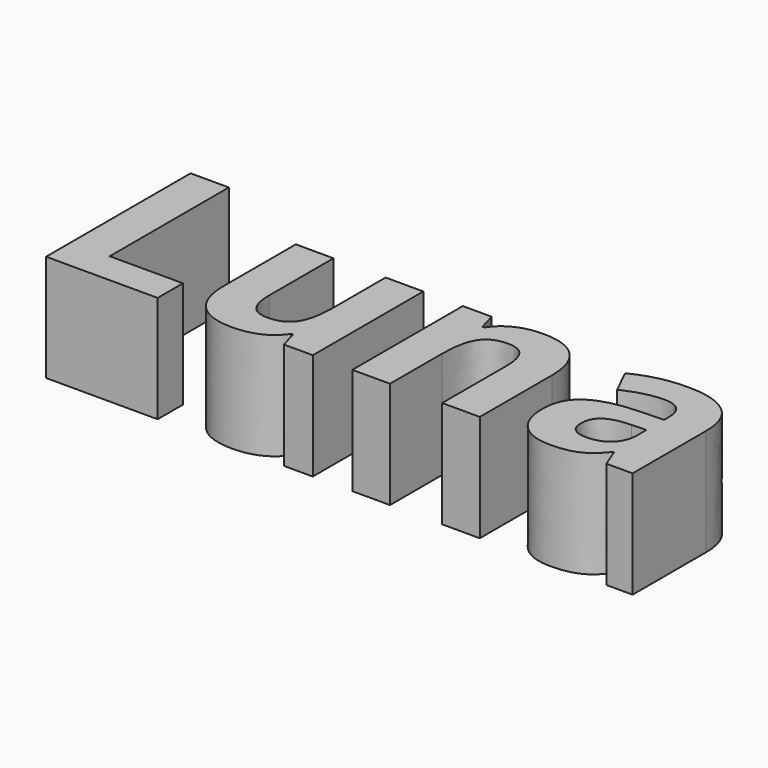
from build123d import *

# Parameters (mm, degrees)
F0_TEXT_SIZE = 60.1547692592
F1_DEPTH     = 25.4


# Not quite as in the source:
# - Text() gives the source's letters only with a copy of the font that has no kerning and outlines rounded to 1/6400 em; it was checked with that copy


with BuildPart() as f1:
    # F0 (on Top) → F1 (new body)
    with BuildSketch(Plane.XY):
        with Locations((-76.9057199359, -21.7394044157)):
            Text('Luna', F0_TEXT_SIZE, font='Open Sans', font_style=FontStyle.BOLD, text_align=(TextAlign.LEFT, TextAlign.BOTTOM))
    extrude(amount=F1_DEPTH)


solid = f1.part
